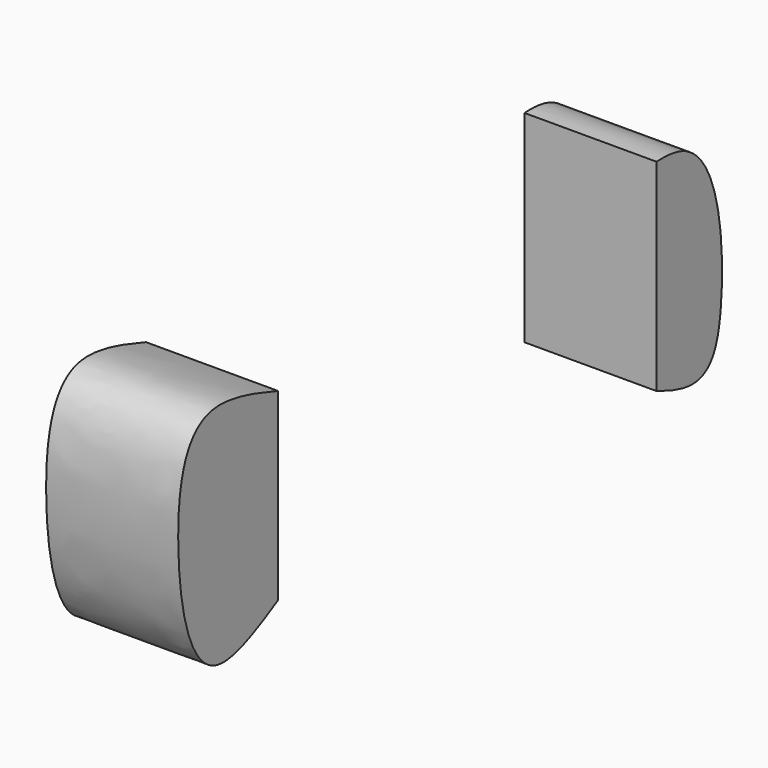
from build123d import *

# Parameters (mm, degrees)
F2_DEPTH = 25.4


with BuildPart() as f2:
    # F1 (on face) → F2 (new body)
    with BuildSketch(Plane.YZ):
        with BuildLine():
            add(Edge.make_bspline(
                [(-42.2480106354, 8.0022732762), (-49.1523837092, 10.4136989063), (-63.8213748972, 14.605450409), (-68.1804772677, -7.7808325222), (-63.6975274058, -31.0515977616), (-56.8205192685, -32.4513763189)],
                knots=[0.7470625357, 0.7470625357, 0.7470625357, 0.7470625357, 0.8057113389, 0.8969839912, 1, 1, 1, 1], degree=3))
            add(Edge.make_bspline(
                [(-56.8205192685, -32.4513763189), (-53.1388638388, -33.2007577684), (-48.1674607533, -30.8149768153), (-42.2480106354, -27.4096912517)],
                knots=[0, 0, 0, 0, 0.0551503562, 0.0551503562, 0.0551503562, 0.0551503562], degree=3))
            Line((-42.2480106354, -27.4096912517), (-42.2480106354, 8.0022732762))
        make_face()
    extrude(amount=F2_DEPTH)


with BuildPart() as f2b:
    # F1 (on face) → F2, piece 2 (new body)
    with BuildSketch(Plane.YZ):
        with BuildLine():
            Line((48.7383008003, 9.8109599666), (48.7383008003, -29.0137173841))
            add(Edge.make_bspline(
                [(48.7383008003, -29.0137173841), (52.2969863828, -30.4945595648), (61.7052048412, -33.3858397255), (65.9289538409, -19.5946219987), (63.3322084855, 8.4877122406), (51.4685517798, 9.9808245247), (48.7383008003, 9.8109599666)],
                knots=[0.2794800975, 0.2794800975, 0.2794800975, 0.2794800975, 0.3139570698, 0.3875541701, 0.4974890007, 0.5252682255, 0.5252682255, 0.5252682255, 0.5252682255], degree=3))
        make_face()
    extrude(amount=F2_DEPTH)


solid = Compound([f2.part, f2b.part])
